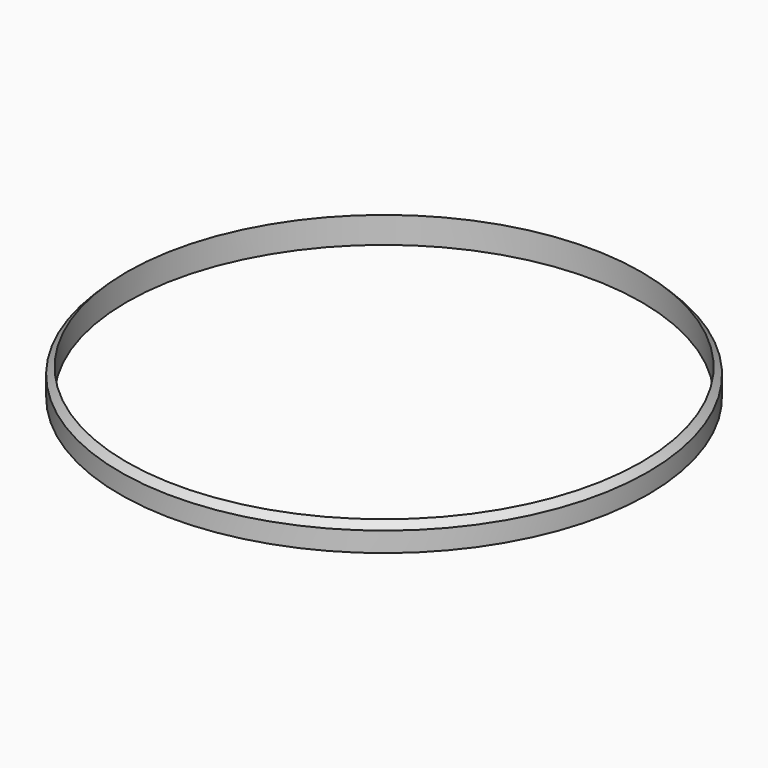
from build123d import *

# Parameters (mm, degrees)
F0_R     = 50.8
F0_R_2   = 49.53
F1_DEPTH = 3.175


# Not quite as in the source:
# - a fillet or chamfer that OpenCascade refuses, or shapes differently, is made with other operations: its cross-section is extruded or revolved along the edge and cut away or added


with BuildPart() as f1:
    # F0 (on Top) → F1 (new body, symmetric)
    with BuildSketch(Plane.XY):
        Circle(F0_R)
        Circle(F0_R_2, mode=Mode.SUBTRACT)
    extrude(amount=F1_DEPTH, both=True)

    # F2: chamfer of 2.54 on 1 edges, made by hand

    # F2_s1 → F2_t2 (revolve, cut)
    with BuildSketch(Plane.XZ):
        Polygon((50.8, 0.635), (48.26, 3.175), (50.8, 3.175), align=None)
    revolve(axis=Axis((0, 0, 3.175), (0, 0, 1)), mode=Mode.SUBTRACT)


solid = f1.part
